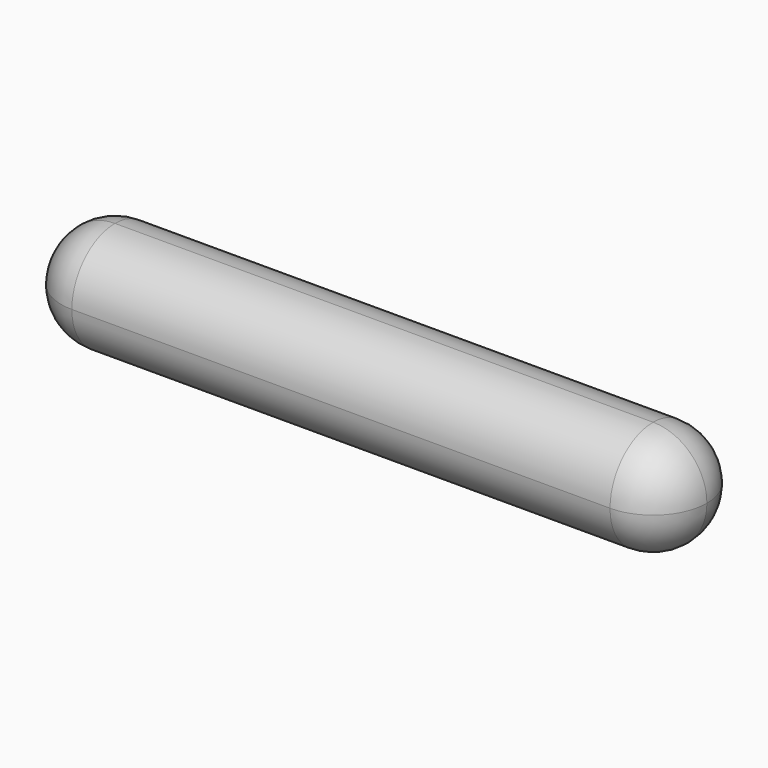
from build123d import *

# Parameters (mm, degrees)
F0_W     = 30
F0_H     = 5
F1_DEPTH = 5
F2_R     = 2.49999


# Not quite as in the source:
# - a fillet or chamfer is up to 0.001 mm smaller than in the source, because OpenCascade refuses the exact size


with BuildPart() as f1:
    # F0 (on Top) → F1 (new body)
    with BuildSketch(Plane.XY):
        Rectangle(F0_W, F0_H)
    extrude(amount=F1_DEPTH)

    # F2 (radius 2.5 in the source; OpenCascade refuses exactly that, so slightly less here)
    f2_edges = [f1.edges().sort_by_distance(p)[0] for p in [
        (0, -2.5, 5),
        (0, 2.5, 5),
        (15, 0, 5),
        (15, 0, 0),
        (15, -2.5, 2.5),
        (-15, 0, 5),
        (0, -2.5, 0),
        (-15, -2.5, 2.5),
        (-15, 0, 0),
        (-15, 2.5, 2.5),
        (0, 2.5, 0),
        (15, 2.5, 2.5),
    ]]
    fillet(f2_edges, radius=F2_R)


solid = f1.part
